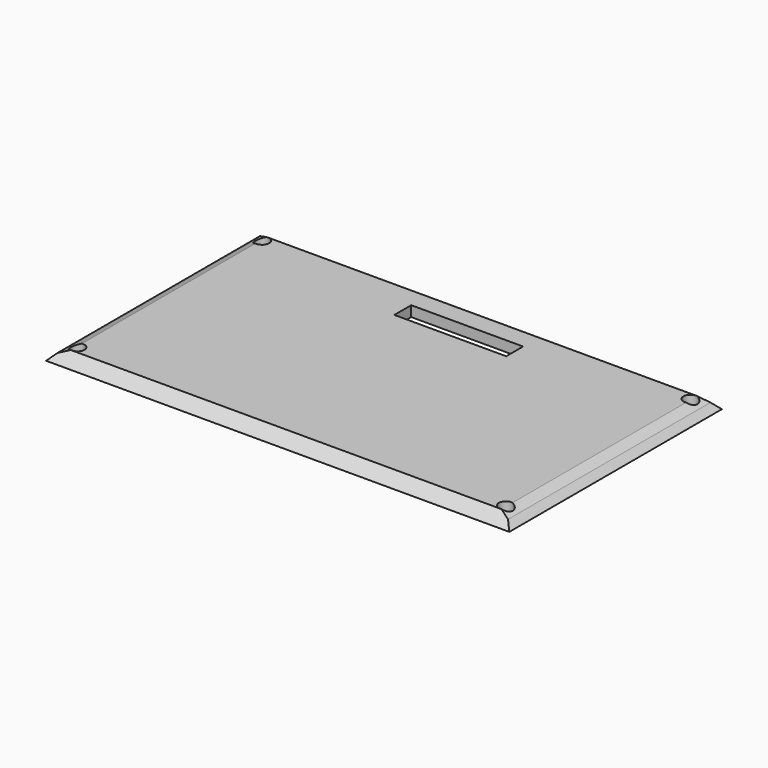
from build123d import *

# Parameters (mm, degrees)
F0_W        = 67.24
F0_H        = 39
F1_DEPTH    = 1.5
F2_T1_DEPTH = 49.2867319519
F3_T1_DEPTH = 73.5267319519
F3_T3_DEPTH = 43.5142834408
F4_R        = 1
F5_DEPTH    = 2
F6_W        = 16
F6_H        = 3.0143252599
F7_DEPTH    = 2


# Not quite as in the source:
# - a fillet or chamfer that OpenCascade refuses, or shapes differently, is made with other operations: its cross-section is extruded or revolved along the edge and cut away or added


with BuildPart() as f1:
    # F0 (on Top) → F1 (new body)
    with BuildSketch(Plane.XY):
        with Locations((12.5632099807, -23.9098862686)):
            Rectangle(F0_W, F0_H)
    extrude(amount=F1_DEPTH)

    # F2: chamfer of 2 on 2 edges, made by hand

    # F2_s2 → F2_t1 (cut)
    with BuildSketch(Plane.XZ.offset(-0.7334797074)):
        Polygon((46.1832099807, -0.5), (44.1832099807, 1.5), (46.1832099807, 1.5), align=None)
        Polygon((-21.0567900193, -0.5), (-19.0567900193, 1.5), (-21.0567900193, 1.5), align=None)
    extrude(amount=F2_T1_DEPTH, mode=Mode.SUBTRACT)

    # F3: chamfer of 2 on 4 edges, made by hand

    # F3_s2 → F3_t1 (cut)
    with BuildSketch(Plane.YZ.offset(-24.2001559952)):
        Polygon((-4.4098862686, -0.5), (-6.4098862686, 1.5), (-4.4098862686, 1.5), align=None)
        Polygon((-41.4098862686, 1.5), (-43.4098862686, -0.5), (-43.4098862686, 1.5), align=None)
    extrude(amount=F3_T1_DEPTH, mode=Mode.SUBTRACT)

    # F3_s4 → F3_t3 (cut)
    with BuildSketch(Plane.XZ.offset(2.1527445482)):
        Polygon((43.354782856, 1.5), (44.7689964183, 0.9142135624), (44.1832099807, 1.5), align=None)
        Polygon((-19.6425764569, 0.9142135624), (-18.2283628946, 1.5), (-19.0567900193, 1.5), align=None)
    extrude(amount=F3_T3_DEPTH, mode=Mode.SUBTRACT)

    # F4 (on face) → F5 (cut)
    with BuildSketch(Plane.XY.offset(1.5)):
        with Locations((43.1832099807, -40.4098862686)):
            Circle(F4_R)
        with Locations((43.1832099807, -7.4098862686)):
            Circle(F4_R)
        with Locations((-18.0567900193, -40.4098862686)):
            Circle(F4_R)
        with Locations((-18.0567900193, -7.4098862686)):
            Circle(F4_R)
    extrude(amount=-F5_DEPTH, mode=Mode.SUBTRACT)

    # F6 (on face) → F7 (cut)
    with BuildSketch(Plane.XY.offset(1.5)):
        with Locations((12.6832099807, -10.7027236386)):
            Rectangle(F6_W, F6_H)
    extrude(amount=-F7_DEPTH, mode=Mode.SUBTRACT)


solid = f1.part
